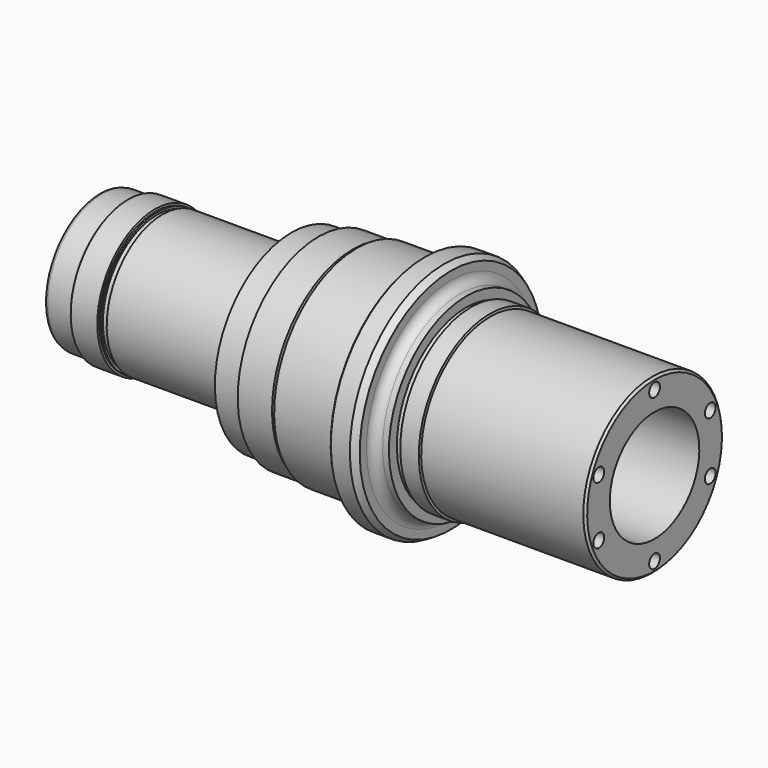
from build123d import *

# Parameters (mm, degrees)
F3_R      = 12.7
F4_R      = 5.08
F6_SIZE   = 3.048
F7_SIZE   = 1.524
F8_R      = 4.5593
F9_DEPTH  = 368.3
F10_R     = 9.5377
F11_DEPTH = 19.05
F12_SIZE2 = 3.1015833811
F12_SIZE  = 1.7907


# Not quite as in the source:
# - a fillet or chamfer that OpenCascade refuses, or shapes differently, is made with other operations: its cross-section is extruded or revolved along the edge and cut away or added
# - a pattern or mirror of a feature is missing from the dataset's text; its kind, count and spacing are read off the source's solid


with BuildPart() as f1:
    # F0 (on Front) → F1 (revolve)
    with BuildSketch(Plane.XZ):
        Polygon((38.1, 96.8375), (0, 96.8375), (0, 87.4649), (25.5470073931, 80.6196), (279.4, 80.6196), (281.2257547563, 79.5655), (526.0414317867, 79.1522667305), (527.9205441475, 77.2668), (606.298, 77.2668), (610.3288152078, 79.1464), (784.098, 79.1464), (784.098, 122.2375), (551.700538686, 122.2375), (550.8498, 125.4125), (524.6542766363, 125.4125), (523.875, 122.5042), (517.525, 122.5042), (517.525, 136.525), (495.935, 136.525), (495.935, 166.6875), (457.9874, 166.6875), (457.9874, 146.05), (362.699461314, 146.05), (357.2002, 142.875), (308.6862, 142.875), (308.6862, 135.636), (270.5862, 135.636), (268.9809399426, 98.8695), (88.0872, 98.8695), (88.0872, 95.6945), (80.1624, 95.6945), (80.1624, 98.8695), (77.724, 98.8695), (76.9923647301, 101.6), (39.376108029, 101.6), align=None)
    revolve(axis=Axis((392.049, 0, 0), (1, 0, 0)))

    # F2: chamfer of 9.525 x 5.499261314 on 1 edges, made by hand

    # F2_s1 → F2_t2 (revolve, cut)
    with BuildSketch(Plane.XZ):
        Polygon((495.935, 161.188238686), (486.41, 166.6875), (495.935, 166.6875), align=None)
    revolve(axis=Axis((495.935, 0, 0), (1, 0, 0)), mode=Mode.SUBTRACT)

    # F3
    f3_edges = [f1.edges().sort_by_distance(p)[0] for p in [
        (495.935, 0, -136.525),
    ]]
    fillet(f3_edges, radius=F3_R)

    # F4
    f4_edges = [f1.edges().sort_by_distance(p)[0] for p in [
        (268.98094, 0, -98.8695),
    ]]
    fillet(f4_edges, radius=F4_R)

    # F5: chamfer of 0.8636 x 3.2229990774 on 2 edges, made by hand

    # F5_s1 → F5_t2 (revolve)
    with BuildSketch(Plane.XZ):
        Polygon((38.1078847952, 96.8669264564), (34.9947067483, 96.8375), (38.1, 96.8375), align=None)
    revolve(axis=Axis((38.1, 0, 0), (1, 0, 0)))

    # F5_s3 → F5_t4 (revolve, cut)
    with BuildSketch(Plane.XZ):
        Polygon((3.2229990774, 96.8375), (0, 95.9739), (0, 96.8375), align=None)
    revolve(axis=Axis((0, 0, 0), (1, 0, 0)), mode=Mode.SUBTRACT)

    # F6
    f6_edges = [f1.edges().sort_by_distance(p)[0] for p in [
        (784.098, 0, -122.2375),
    ]]
    chamfer(f6_edges, length=F6_SIZE)

    # F7
    f7_edges = [f1.edges().sort_by_distance(p)[0] for p in [
        (457.9874, 0, -166.6875),
    ]]
    chamfer(f7_edges, length=F7_SIZE)

    # F8 (on face) → F9 (cut)
    with BuildSketch(Plane.YZ.offset(784.098)):
        with Locations((0, 106.68)):
            Circle(F8_R)
        with Locations((0, -106.68)):
            Circle(F8_R)
        with Locations((98.5178773125, 40.9249343291)):
            Circle(F8_R)
        with Locations((98.5594685283, -40.8246685647)):
            Circle(F8_R)
        with Locations((-98.5594685283, -40.8246685647)):
            Circle(F8_R)
        with Locations((-98.5568319807, 40.8310331723)):
            Circle(F8_R)
    extrude(amount=-F9_DEPTH, mode=Mode.SUBTRACT)

    # F10 (on face) → F11 (cut)
    with BuildSketch(Plane.YZ.offset(784.098)):
        with Locations((98.5178773125, 40.9249343291)):
            Circle(F10_R)
        with Locations((0, 106.68)):
            Circle(F10_R)
        with Locations((-98.5568319807, 40.8310331723)):
            Circle(F10_R)
        with Locations((-98.5594685283, -40.8246685647)):
            Circle(F10_R)
        with Locations((98.5594685283, -40.8246685647)):
            Circle(F10_R)
        with Locations((0, -106.68)):
            Circle(F10_R)
    extrude(amount=-F11_DEPTH, mode=Mode.SUBTRACT)

    # F12
    f12_edges = [f1.edges().sort_by_distance(p)[0] for p in [
        (765.048, -4.5593, 106.68),
        (765.048, -103.116132, 40.831033),
        (765.048, -4.5593, -106.68),
        (765.048, -103.118769, -40.824669),
        (765.048, 94.000169, -40.824669),
        (765.048, 93.958577, 40.924934),
    ]]
    chamfer(f12_edges, length=F12_SIZE, length2=F12_SIZE2)

    # F13 (on Front) → F14 (revolve, cut)
    with BuildSketch(Plane.XZ):
        Polygon((422.798187933, 106.3411877659), (269.5992007246, 113.03), (264.7598683834, 110.7791513205), (264.7598683834, 103.5775052515), (269.1864958911, 103.5775052515), (288.2183645122, 102.7465559222), (288.354086236, 105.8550944636), (290.9651204006, 107.5335002234), (420.9986925125, 101.8561118552), align=None)
    f14 = revolve(axis=Axis((346.1986943288, 0, 109.6855938829), (0.9990482216, 0, -0.0436193874)), mode=Mode.SUBTRACT)

    # F14_copies: F14 across plane
    add(f14.mirror(Plane(origin=(0, 0, -1e-06), x_dir=(-1, 0, 0), z_dir=(0, 0, -1))), mode=Mode.SUBTRACT)


solid = f1.part
